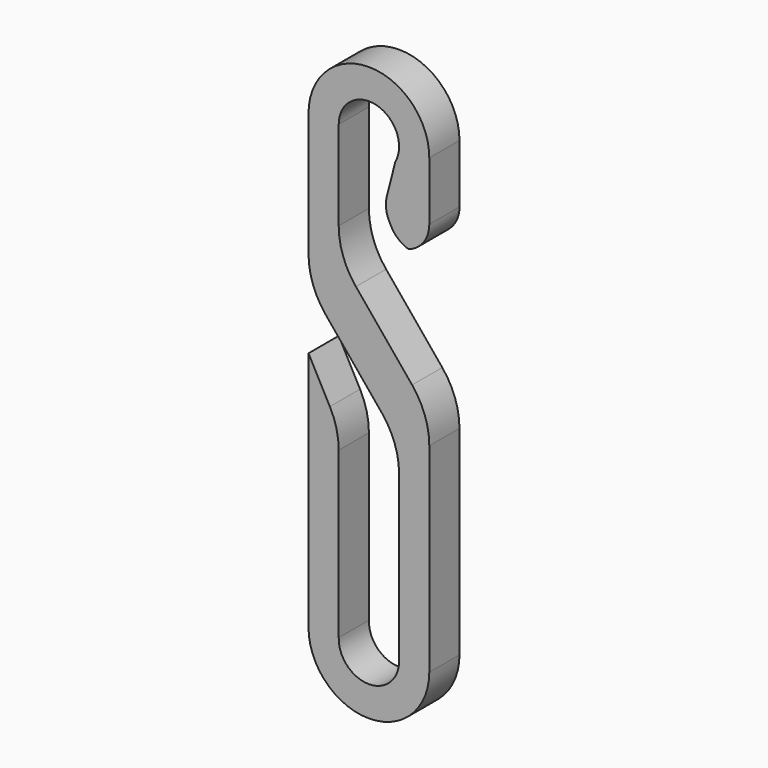
from build123d import *

# Parameters (mm, degrees)
F1_DEPTH    = 2.5
F2_R        = 5
F3_T1_DEPTH = 6.2430809658
F3_T3_DEPTH = 8.6803398875
F3_T5_DEPTH = 12.5


# Not quite as in the source:
# - a fillet or chamfer that OpenCascade refuses, or shapes differently, is made with other operations: its cross-section is extruded or revolved along the edge and cut away or added


with BuildPart() as f1:
    # F0 (on Front) → F1 (new body)
    with BuildSketch(Plane.XZ):
        with BuildLine():
            ThreePointArc((-2, 0), (0.5, 1.9364916731), (1.75, -0.9682458366))
            Line((1.75, -0.9682458366), (1, -3.8729833462))
            Line((1, -3.8729833462), (2, -5.8729833462))
            Line((2, -5.8729833462), (4, -5.8729833462))
            Line((4, -5.8729833462), (4, 0))
            ThreePointArc((4, 0), (0, 4), (-4, 0))
            Line((-4, 0), (-4, -10))
            Line((-4, -10), (2, -17.2908526251))
            Line((2, -17.2908526251), (2, -30))
            ThreePointArc((2, -30), (-0.0346553957, -31.9996997283), (-1.9987990036, -29.9306996147))
            Line((-1.9987990036, -29.9306996147), (-1.9987990036, -17.7522518683))
            Line((-1.9987990036, -17.7522518683), (-4, -14))
            Line((-4, -14), (-4, -30))
            ThreePointArc((-4, -30), (0, -34), (4, -30))
            Line((4, -30), (4, -15))
            Line((4, -15), (-2, -7.7091473749))
            Line((-2, -7.7091473749), (-2, 0))
        make_face()
    extrude(amount=F1_DEPTH)

    # F2
    f2_edges = [f1.edges().sort_by_distance(p)[0] for p in [
        (-4, -1.25, -10),
        (2, -1.25, -17.290853),
        (4, -1.25, -15),
        (-2, -1.25, -7.709147),
        (-1.998799, -1.25, -17.752252),
    ]]
    fillet(f2_edges, radius=F2_R)

    # F3: fillet of radius 2 on 3 edges, made by hand

    # F3_s2 → F3_t1 (cut)
    with BuildSketch(Plane.XZ.offset(-1.8715404829)):
        with BuildLine():
            ThreePointArc((1.1871540483, -3.148138834), (1.1347622142, -3.8587151733), (1.3347913394, -4.542566025))
            Line((1.3347913394, -4.542566025), (1, -3.8729833462))
            Line((1, -3.8729833462), (1.1871540483, -3.148138834))
        make_face()
    extrude(amount=F3_T1_DEPTH, mode=Mode.SUBTRACT)

    # F3_s4 → F3_t3 (cut)
    with BuildSketch(Plane.XZ.offset(-3.0901699437)):
        with BuildLine():
            ThreePointArc((1.4472135955, -4.7674105372), (2.1846057533, -5.5742849629), (3.2360679775, -5.8729833462))
            Line((3.2360679775, -5.8729833462), (2, -5.8729833462))
            Line((2, -5.8729833462), (1.4472135955, -4.7674105372))
        make_face()
    extrude(amount=F3_T3_DEPTH, mode=Mode.SUBTRACT)

    # F3_s6 → F3_t5 (cut)
    with BuildSketch(Plane.XZ.offset(-5)):
        with BuildLine():
            ThreePointArc((2, -5.8729833462), (3.4142135624, -5.2871969086), (4, -3.8729833462))
            Line((4, -3.8729833462), (4, -5.8729833462))
            Line((4, -5.8729833462), (2, -5.8729833462))
        make_face()
    extrude(amount=F3_T5_DEPTH, mode=Mode.SUBTRACT)


solid = f1.part
